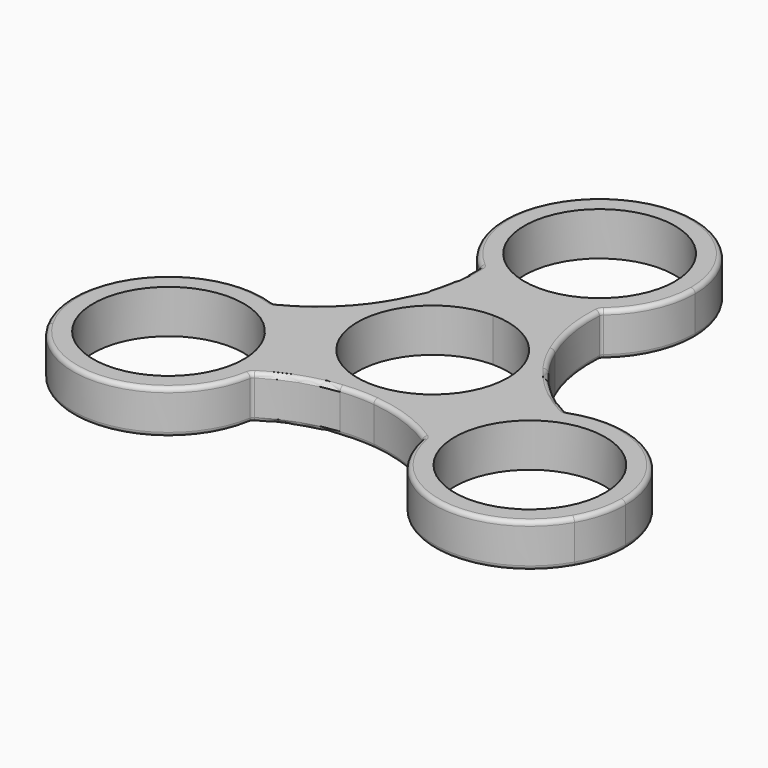
from build123d import *

# Parameters (mm, degrees)
F0_R     = 10.9982
F1_DEPTH = 6.35
F2_R     = 0.635


with BuildPart() as f1:
    # F0 (on Top) → F1 (new body)
    with BuildSketch(Plane.XY):
        with BuildLine():
            ThreePointArc((13.97, 30.48), (9.8782816978, 40.3582817686), (-1.001e-07, 44.45))
            ThreePointArc((-1.001e-07, 44.45), (-13.1905941087, 35.0809919648), (-8.6885924199, 19.5406553322))
            ThreePointArc((-8.6885924199, 19.5406553322), (-4.6009920121, 17.2894059078), (0, 16.51))
            ThreePointArc((0, 16.51), (4.7049878122, 17.3261416426), (8.8602352549, 19.6792069167))
            ThreePointArc((8.8602352549, 19.6792069167), (12.6281112307, 24.5057463441), (13.97, 30.48))
        make_face()
        with BuildLine():
            ThreePointArc((10.9982, 30.48), (7.7769018008, 22.7030981992), (0, 19.4818))
            ThreePointArc((0, 19.4818), (-7.7769018008, 38.2569018008), (10.9982, 30.48))
        make_face(mode=Mode.SUBTRACT)
        with BuildLine():
            ThreePointArc((12.6125754888, -17.5127922726), (23.8941639919, -28.984069382), (38.4948290898, -22.2250001877))
            ThreePointArc((38.4948290898, -22.2250001877), (39.8904380726, -18.8557021648), (40.3664543073, -15.24))
            ThreePointArc((40.3664543073, -15.24), (34.2546482856, -3.6896888614), (21.2670001342, -2.2457859074))
            ThreePointArc((21.2670001342, -2.2457859074), (14.2433101852, -8.3507338601), (12.6125754888, -17.5127922726))
        make_face()
        with Locations((26.3964543073, -15.24)):
            Circle(F0_R, mode=Mode.SUBTRACT)
        with BuildLine():
            ThreePointArc((-21.4728107437, -2.1664146441), (-37.0480222865, -6.2009182111), (-38.4948294602, -22.2249995463))
            ThreePointArc((-38.4948294602, -22.2249995463), (-23.7857334836, -28.9638856298), (-12.5784077143, -17.2948694248))
            ThreePointArc((-12.5784077143, -17.2948694248), (-12.4644944505, -16.2702400437), (-12.4264543073, -15.24))
            ThreePointArc((-12.4264543073, -15.24), (-14.9085432574, -7.2908617003), (-21.4728107437, -2.1664146441))
        make_face()
        with Locations((-26.3964543073, -15.24)):
            Circle(F0_R, mode=Mode.SUBTRACT)
        with BuildLine():
            ThreePointArc((0, 13.97), (-5.856417794, 12.6831885038), (-10.6339371279, 9.0598168392))
            ThreePointArc((-10.6339371279, 9.0598168392), (-11.7632136635, 6.8551872307), (-13.1246525512, 4.7858536762))
            ThreePointArc((-13.1246525512, 4.7858536762), (-12.126574558, -6.9359274426), (-2.5290629724, -13.7391681146))
            ThreePointArc((-2.5290629724, -13.7391681146), (-0.0551594577, -13.6148354781), (2.4176554132, -13.7592093633))
            ThreePointArc((2.4176554132, -13.7592093633), (10.6989613076, -8.9829353186), (13.97, 0))
            ThreePointArc((13.97, 0), (13.7667717966, 2.3742144594), (13.1630001003, 4.6793512754))
            ThreePointArc((13.1630001003, 4.6793512754), (11.8183731212, 6.7596482474), (10.706997138, 8.9733556871))
            ThreePointArc((10.706997138, 8.9733556871), (5.9077542709, 12.6593577829), (0, 13.97))
        make_face()
        with BuildLine():
            ThreePointArc((10.9982, 0), (-7.7769018008, -7.7769018008), (0, 10.9982))
            ThreePointArc((0, 10.9982), (7.7769018008, 7.7769018008), (10.9982, 0))
        make_face(mode=Mode.SUBTRACT)
        with BuildLine():
            ThreePointArc((0, 16.51), (-4.6009920121, 17.2894059078), (-8.6885924199, 19.5406553322))
            ThreePointArc((-8.6885924199, 19.5406553322), (-9.0410842982, 14.185124608), (-10.6339371279, 9.0598168392))
            ThreePointArc((-10.6339371279, 9.0598168392), (-5.856417794, 12.6831885038), (0, 13.97))
            Line((0, 13.97), (0, 16.51))
        make_face()
        with BuildLine():
            ThreePointArc((10.706997138, 8.9733556871), (9.1376356479, 14.2148495037), (8.8602352549, 19.6792069167))
            ThreePointArc((8.8602352549, 19.6792069167), (4.7049878122, 17.3261416426), (0, 16.51))
            Line((0, 16.51), (0, 13.97))
            ThreePointArc((0, 13.97), (5.9077542709, 12.6593577829), (10.706997138, 8.9733556871))
        make_face()
        with BuildLine():
            ThreePointArc((2.4176554132, -13.7592093633), (7.7416029572, -15.0208493535), (12.6125754888, -17.5127922726))
            ThreePointArc((12.6125754888, -17.5127922726), (14.2433101852, -8.3507338601), (21.2670001342, -2.2457859074))
            ThreePointArc((21.2670001342, -2.2457859074), (16.8052204155, 0.737246376), (13.1630001003, 4.6793512754))
            ThreePointArc((13.1630001003, 4.6793512754), (13.7667717966, 2.3742144594), (13.97, 0))
            ThreePointArc((13.97, 0), (10.6989613076, -8.9829353186), (2.4176554132, -13.7592093633))
        make_face()
        with BuildLine():
            ThreePointArc((-13.1246525512, 4.7858536762), (-16.8792386051, 0.8059998498), (-21.4728107437, -2.1664146441))
            ThreePointArc((-21.4728107437, -2.1664146441), (-14.9085432574, -7.2908617003), (-12.4264543073, -15.24))
            ThreePointArc((-12.4264543073, -15.24), (-12.4644944505, -16.2702400437), (-12.5784077143, -17.2948694248))
            ThreePointArc((-12.5784077143, -17.2948694248), (-7.7641361173, -14.922370984), (-2.5290629724, -13.7391681146))
            ThreePointArc((-2.5290629724, -13.7391681146), (-12.126574558, -6.9359274426), (-13.1246525512, 4.7858536762))
        make_face()
    extrude(amount=F1_DEPTH)

    # F2
    f2_edges = [f1.edges().sort_by_distance(p)[0] for p in [
        (11.766443, 6.850928, 6.35),
        (-11.816299, 6.764575, 6.35),
        (-11.816299, 6.764575, 0),
        (11.766443, 6.850928, 0),
        (0.049856, -13.615502, 0),
        (8.860235, 19.679207, 3.175),
        (-8.688592, 19.540655, 3.175),
        (-0.110293, 44.449565, 0),
        (-0.110293, 44.449565, 6.35),
        (12.612575, -17.512792, 3.175),
        (21.267, -2.245786, 3.175),
        (38.549598, -22.129266, 0),
        (38.549598, -22.129266, 6.35),
        (-21.472811, -2.166415, 3.175),
        (-12.578408, -17.294869, 3.175),
        (-38.439306, -22.320298, 0),
        (-38.439306, -22.320298, 6.35),
        (0.049856, -13.615502, 6.35),
    ]]
    fillet(f2_edges, radius=F2_R)


solid = f1.part
